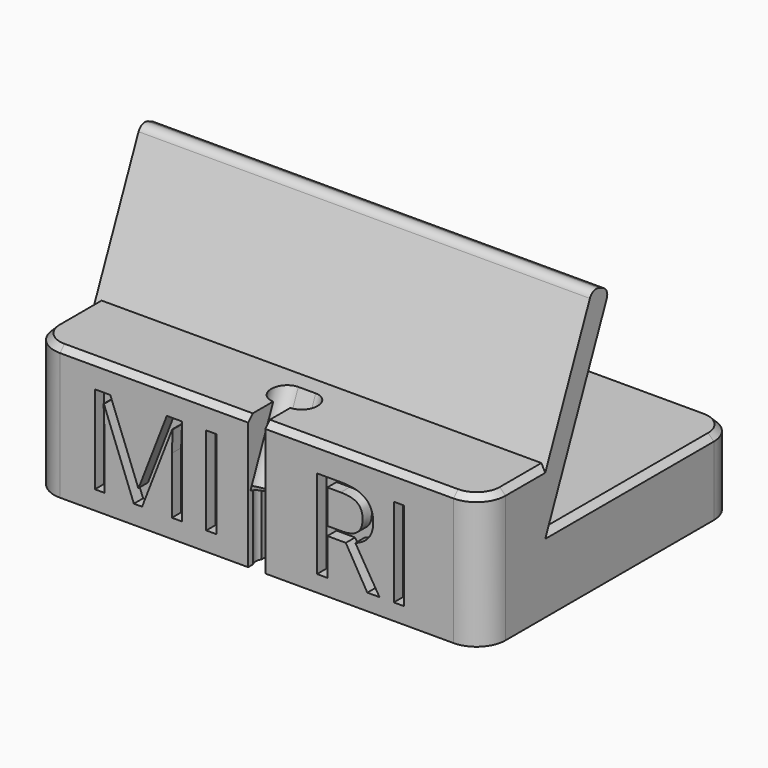
from build123d import *

# Parameters (mm, degrees)
F1_DEPTH        = 50
F3_DEPTH        = 78.001
F4_R            = 1.5
F6_DEPTH        = 48
F7_W            = 2.9618441971
F7_H            = 23
F8_DEPTH        = 7
F9_R            = 1.75
F10_DEPTH       = 12
F12_DEPTH       = 40.9
F13_SIZE        = 5
F14_SIZE        = 1
F15_TEXT_SIZE   = 21.3189121698
F15_TEXT_SIZE_2 = 21.4610391089
F16_DEPTH       = 2


# Not quite as in the source:
# - ends of sketch curves that miss each other by under 0.0002 mm in the source are joined
# - Text() gives the source's letters only with a copy of the font that has no kerning and outlines rounded to 1/6400 em; it was checked with that copy


with BuildPart() as f1:
    # F0 (on Top) → F1 (new body)
    with BuildSketch(Plane.XY):
        with BuildLine():
            Line((34, 27.5), (-34, 27.5))
            ThreePointArc((-34, 27.5), (-37.5355339059, 26.0355339059), (-39, 22.5))
            Line((-39, 22.5), (-39, -22.5))
            ThreePointArc((-39, -22.5), (-37.5355339059, -26.0355339059), (-34, -27.5))
            Line((-34, -27.5), (34, -27.5))
            ThreePointArc((34, -27.5), (37.5355339059, -26.0355339059), (39, -22.5))
            Line((39, -22.5), (39, 22.5))
            ThreePointArc((39, 22.5), (37.5355339059, 26.0355339059), (34, 27.5))
        make_face()
    extrude(amount=F1_DEPTH)

    # F2 (on face) → F3 (cut, through all)
    with BuildSketch(Plane.YZ.offset(39)):
        Polygon((-27.5, 50), (-27.5, 23), (-13.5, 23), (-3.6840454403, 45.992325591), (-0.054631016, 44.4428447903), (-13.5, 12.9491882652), (27.5, 12.9491882652), (27.5, 50), align=None)
    extrude(amount=-F3_DEPTH, mode=Mode.SUBTRACT)

    # F4
    f4_edges = [f1.edges().sort_by_distance(p)[0] for p in [
        (0, -3.684045, 45.992326),
        (0, -0.054631, 44.442845),
    ]]
    fillet(f4_edges, radius=F4_R)

    # F5 (on face) → F6 (cut)
    with BuildSketch(Plane(origin=(0, 27.5, 0), x_dir=(-1, 0, 0), z_dir=(0, 1, 0))):
        with BuildLine():
            Line((1.4809220986, 2.2615262321), (1.5, 2.5))
            ThreePointArc((1.5, 2.5), (0, 4), (-1.5, 2.5))
            Line((-1.5, 2.5), (-1.4809220986, 2.2615262321))
            ThreePointArc((-1.4809220986, 2.2615262321), (0, 1), (1.4809220986, 2.2615262321))
        make_face()
        with BuildLine():
            ThreePointArc((1.4809220986, 2.2615262321), (1.4952229178, 2.3803821666), (1.5, 2.5))
            Line((1.5, 2.5), (1.4809220986, 2.2615262321))
        make_face()
        with BuildLine():
            Line((-1.4809220986, 2.2615262321), (-1.5, 2.5))
            ThreePointArc((-1.5, 2.5), (-1.4952229178, 2.3803821666), (-1.4809220986, 2.2615262321))
        make_face()
        with BuildLine():
            Line((1.3, 0), (1.4809220986, 2.2615262321))
            ThreePointArc((1.4809220986, 2.2615262321), (0, 1), (-1.4809220986, 2.2615262321))
            Line((-1.4809220986, 2.2615262321), (-1.3, 0))
            Line((-1.3, 0), (1.3, 0))
        make_face()
    extrude(amount=-F6_DEPTH, mode=Mode.SUBTRACT)

    # F7 (on face) → F8 (cut)
    with BuildSketch(Plane.XZ.offset(27.5)):
        with Locations((0, 11.5)):
            Rectangle(F7_W, F7_H)
    extrude(amount=-F8_DEPTH, mode=Mode.SUBTRACT)

    # F9 (on face) → F10 (cut)
    with BuildSketch(Plane(origin=(0, 0, 0), x_dir=(1, 0, 0), z_dir=(0, 0, -1))):
        with Locations((0, 25.5)):
            Circle(F9_R)
    extrude(amount=-F10_DEPTH, mode=Mode.SUBTRACT)

    # F11 (on face) → F12 (cut)
    with BuildSketch(Plane(origin=(0, 16.0401822737, 37.5715974571), x_dir=(1, 0, 0), z_dir=(0, 0.3926381824, 0.9196930236))):
        with BuildLine():
            ThreePointArc((1.5000002555, -29.322236345), (3.2677672085, -28.590003298), (4.0000002555, -26.822236345))
            ThreePointArc((4.0000002555, -26.822236345), (3.2677672085, -25.0544693921), (1.5000002555, -24.322236345))
            ThreePointArc((1.5000002555, -24.322236345), (0.7094308404, -24.4505280999), (2.555e-07, -24.822236345))
            ThreePointArc((2.555e-07, -24.822236345), (0.736068233, -25.7042023563), (1.0000002555, -26.822236345))
            ThreePointArc((1.0000002555, -26.822236345), (0.7360682059, -27.9402703879), (1.586e-07, -28.8222364177))
            ThreePointArc((1.586e-07, -28.8222364177), (0.709430783, -29.193944571), (1.5000002555, -29.322236345))
        make_face()
        with BuildLine():
            ThreePointArc((2.555e-07, -24.822236345), (0.7094308404, -24.4505280999), (1.5000002555, -24.322236345))
            Line((1.5000002555, -24.322236345), (-1.5000002555, -24.322236345))
            ThreePointArc((-1.5000002555, -24.322236345), (-0.7094305718, -24.4505280191), (2.555e-07, -24.822236345))
        make_face()
        with BuildLine():
            Line((0, -29.322236345), (1.5000002555, -29.322236345))
            ThreePointArc((1.5000002555, -29.322236345), (0.709430783, -29.193944571), (1.586e-07, -28.8222362724))
            Line((1.586e-07, -28.8222362724), (0, -29.322236345))
        make_face()
        with BuildLine():
            ThreePointArc((1.586e-07, -28.8222362724), (-0.9999997445, -26.8222362845), (2.555e-07, -24.822236345))
            ThreePointArc((2.555e-07, -24.822236345), (-0.7094305718, -24.4505280191), (-1.5000002555, -24.322236345))
            ThreePointArc((-1.5000002555, -24.322236345), (-3.9999997445, -26.822236345), (-1.5000002555, -29.322236345))
            ThreePointArc((-1.5000002555, -29.322236345), (-0.7094306293, -29.1939446901), (1.586e-07, -28.8222362724))
        make_face()
        with BuildLine():
            Line((0, -29.322236345), (2.84e-08, -28.822236345))
            ThreePointArc((2.84e-08, -28.822236345), (-0.7094306293, -29.1939446901), (-1.5000002555, -29.322236345))
            Line((-1.5000002555, -29.322236345), (0, -29.322236345))
        make_face()
        with BuildLine():
            ThreePointArc((1.0000002555, -26.822236345), (0.736068233, -25.7042023563), (2.555e-07, -24.822236345))
            Line((2.555e-07, -24.822236345), (2.84e-08, -28.822236345))
            ThreePointArc((2.84e-08, -28.822236345), (0.7360682059, -27.9402703879), (1.0000002555, -26.822236345))
        make_face()
        with BuildLine():
            Line((2.84e-08, -28.822236345), (2.555e-07, -24.822236345))
            ThreePointArc((2.555e-07, -24.822236345), (-0.9999997445, -26.8222362845), (2.84e-08, -28.822236345))
        make_face()
    extrude(amount=-F12_DEPTH, mode=Mode.SUBTRACT)

    # F13
    f13_edges = [f1.edges().sort_by_distance(p)[0] for p in [
        (0, -20.5, 4),
    ]]
    chamfer(f13_edges, length=F13_SIZE)

    # F14
    f14_edges = [f1.edges().sort_by_distance(p)[0] for p in [
        (-39, 4.5, 12.949188),
        (39, -18, 23),
        (-17.740461, -27.5, 23),
        (-39, -18, 23),
        (-37.535534, -26.035534, 23),
        (17.740461, -27.5, 23),
        (37.535534, -26.035534, 23),
        (0, 27.5, 12.949188),
        (-37.535534, 26.035534, 12.949188),
        (39, 4.5, 12.949188),
        (37.535534, 26.035534, 12.949188),
    ]]
    chamfer(f14_edges, length=F14_SIZE)

    # F15 (on face) → F16 (cut)
    with BuildSketch(Plane.XZ.offset(27.5)):
        with Locations((-30.0560276955, 3.2392996363)):
            Text('MI', F15_TEXT_SIZE, font='Open Sans', text_align=(TextAlign.LEFT, TextAlign.BOTTOM))
        with Locations((8.3180139773, 2.8299773112)):
            Text('RI', F15_TEXT_SIZE_2, font='Open Sans', text_align=(TextAlign.LEFT, TextAlign.BOTTOM))
    extrude(amount=-F16_DEPTH, mode=Mode.SUBTRACT)


solid = f1.part
